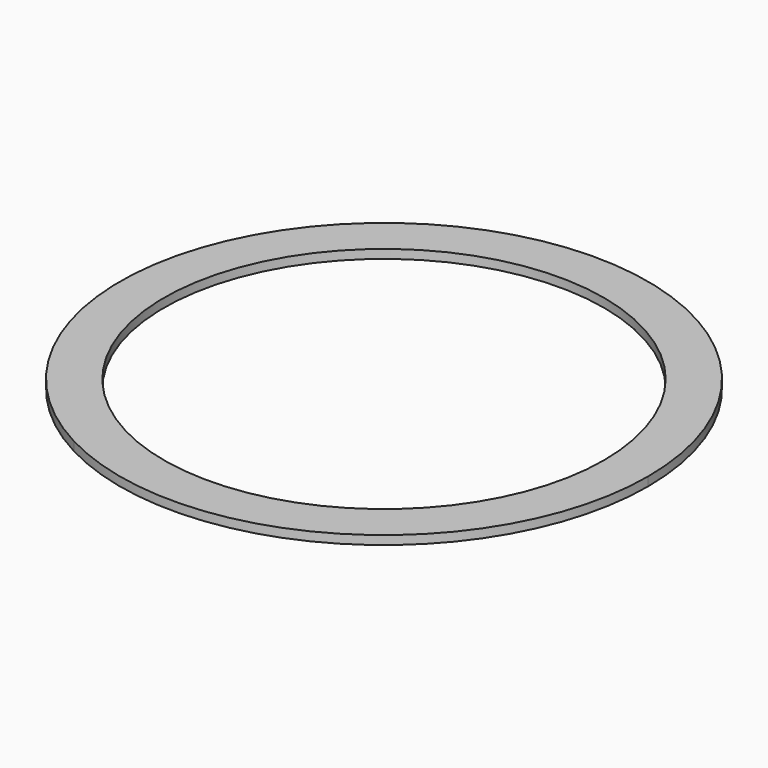
from build123d import *

# Parameters (mm, degrees)
F1_R     = 0.276
F2_DEPTH = 0.3
F1_R_2   = 0.25


# Not quite as in the source:
# - a feature of the source that left no trace in its solid (it failed there, or was rolled back) is left out


with BuildPart() as f2:
    # F1 (on face) → F2 (new body)
    with BuildSketch(Plane.XY):
        with Locations((-3.8761778269, -7.2584804147)):
            Circle(F1_R)
    extrude(amount=F2_DEPTH)


with BuildPart() as f2b:
    # F1 (on face) → F2, piece 2 (new body)
    with BuildSketch(Plane.XY):
        with Locations((0.2459411263, -8.2172408689)):
            Circle(F1_R_2)
    extrude(amount=F2_DEPTH)


with BuildPart() as f2c:
    # F0 (on Top) → F2, piece 3 (new body)
    with BuildSketch(Plane.XY):
        with BuildLine():
            ThreePointArc((-4.2041171366, -7.9577257494), (4.6455863877, -7.7083413984), (9, 0))
            ThreePointArc((9, 0), (-4.6455863877, 7.7083413984), (-4.2041171366, -7.9577257494))
        make_face()
        with BuildLine():
            ThreePointArc((7.5, 0), (3.8713219897, -6.423617832), (-3.5034309471, -6.6314381245))
            ThreePointArc((-3.5034309471, -6.6314381245), (-3.8713219897, 6.423617832), (7.5, 0))
        make_face(mode=Mode.SUBTRACT)
    extrude(amount=F2_DEPTH)


solid = Compound([f2.part, f2b.part, f2c.part])
